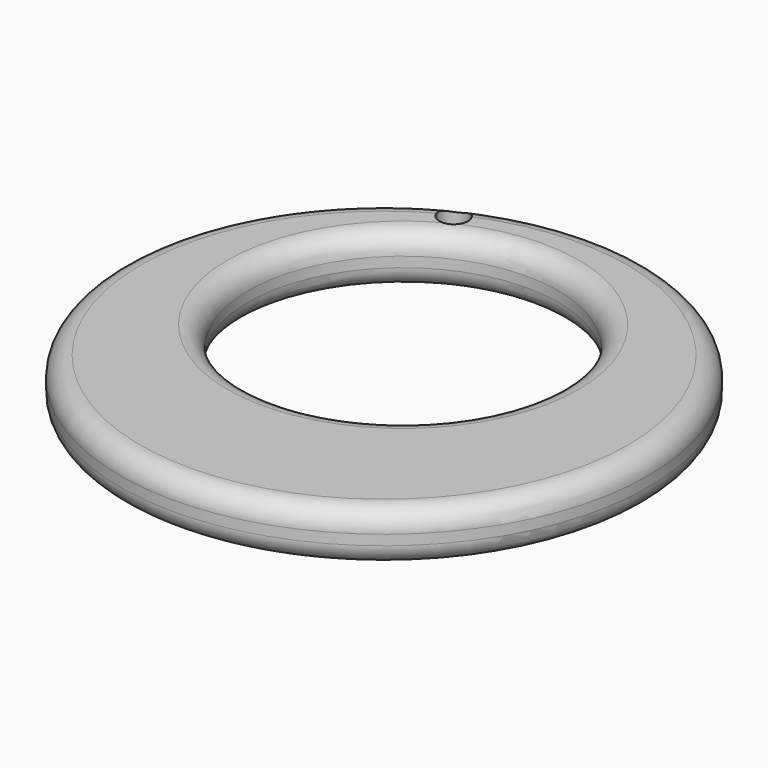
from build123d import *

# Parameters (mm, degrees)
F0_R     = 26
F0_R_2   = 15.2795824113
F0_R_3   = 1.4029986266
F1_DEPTH = 5


# Not quite as in the source:
# - a fillet or chamfer that OpenCascade refuses, or shapes differently, is made with other operations: its cross-section is extruded or revolved along the edge and cut away or added


with BuildPart() as f1:
    # F0 (on Top) → F1 (new body)
    with BuildSketch(Plane.XY):
        with Locations((-44.8659136891, 39.1403473914)):
            Circle(F0_R)
        with Locations((-46.8892939389, 44.0070107579)):
            Circle(F0_R_2, mode=Mode.SUBTRACT)
        with Locations((-55.1761128008, 60.6025718153)):
            Circle(F0_R_3, mode=Mode.SUBTRACT)
    extrude(amount=F1_DEPTH)

    # F2: fillet of radius 2 on 4 edges, made by hand

    # F2_s1 → F2_t2 (revolve, cut)
    with BuildSketch(Plane.XZ.offset(-39.1403473914)):
        with BuildLine():
            ThreePointArc((-18.8659136891, 3), (-19.4517001268, 4.4142135624), (-20.8659136891, 5))
            Line((-20.8659136891, 5), (-18.8659136891, 5))
            Line((-18.8659136891, 5), (-18.8659136891, 3))
        make_face()
    revolve(axis=Axis((-44.8659136891, 39.1403473914, 5), (0, 0, 1)), mode=Mode.SUBTRACT)

    # F2_s3 → F2_t4 (revolve, cut)
    with BuildSketch(Plane.XZ.offset(-39.1403473914)):
        with BuildLine():
            ThreePointArc((-18.8659136891, 2), (-19.4517001268, 0.5857864376), (-20.8659136891, 0))
            Line((-20.8659136891, 0), (-18.8659136891, 0))
            Line((-18.8659136891, 0), (-18.8659136891, 2))
        make_face()
    revolve(axis=Axis((-44.8659136891, 39.1403473914, 0), (0, 0, 1)), mode=Mode.SUBTRACT)

    # F2_s5 → F2_t6 (revolve, cut)
    with BuildSketch(Plane.XZ.offset(-44.0070107579)):
        with BuildLine():
            ThreePointArc((-31.6097115275, 3), (-31.0239250899, 4.4142135624), (-29.6097115275, 5))
            Line((-29.6097115275, 5), (-31.6097115275, 5))
            Line((-31.6097115275, 5), (-31.6097115275, 3))
        make_face()
    revolve(axis=Axis((-46.8892939389, 44.0070107579, 5), (0, 0, 1)), mode=Mode.SUBTRACT)

    # F2_s7 → F2_t8 (revolve, cut)
    with BuildSketch(Plane.XZ.offset(-44.0070107579)):
        with BuildLine():
            ThreePointArc((-31.6097115275, 2), (-31.0239250899, 0.5857864376), (-29.6097115275, 0))
            Line((-29.6097115275, 0), (-31.6097115275, 0))
            Line((-31.6097115275, 0), (-31.6097115275, 2))
        make_face()
    revolve(axis=Axis((-46.8892939389, 44.0070107579, 0), (0, 0, 1)), mode=Mode.SUBTRACT)


solid = f1.part
